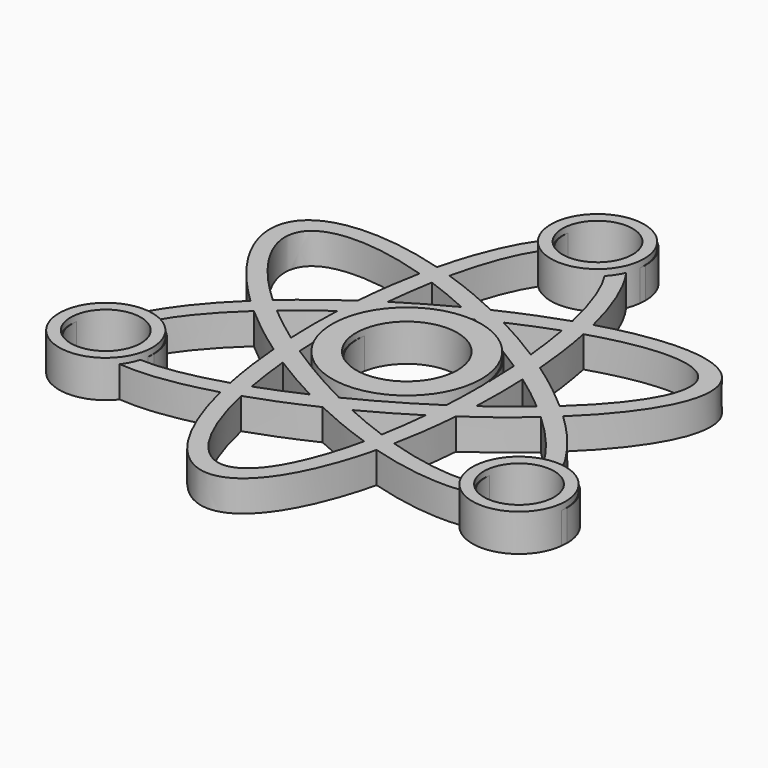
from build123d import *

# Parameters (mm, degrees)
F1_R     = 12
F1_R_2   = 8.15
F2_DEPTH = 6
F1_R_3   = 7.5
F1_R_4   = 5.65
F0_R     = 8.15
F0_R_2   = 5.65
F3_DEPTH = 5


with BuildPart() as f2:
    # F1 (on Top) → F2 (new body)
    with BuildSketch(Plane.XY):
        Circle(F1_R)
        Circle(F1_R_2, mode=Mode.SUBTRACT)
    extrude(amount=F2_DEPTH)


with BuildPart() as f2b:
    # F1 (on Top) → F2, piece 2 (new body)
    with BuildSketch(Plane.XY):
        with Locations((-33.1374317474, -19.1319051396)):
            Circle(F1_R_3)
        with Locations((-33.1374317474, -19.1319051396)):
            Circle(F1_R_4, mode=Mode.SUBTRACT)
    extrude(amount=F2_DEPTH)


with BuildPart() as f2c:
    # F1 (on Top) → F2, piece 3 (new body)
    with BuildSketch(Plane.XY):
        with Locations((33.5652192555, -19.3788883726)):
            Circle(F1_R_3)
        with Locations((33.5652192555, -19.3788883726)):
            Circle(F1_R_4, mode=Mode.SUBTRACT)
    extrude(amount=F2_DEPTH)


with BuildPart() as f2d:
    # F1 (on Top) → F2, piece 4 (new body)
    with BuildSketch(Plane.XY):
        with Locations((0.0270425226, 38.3360795677)):
            Circle(F1_R_3)
        with Locations((0.0270425226, 38.3360795677)):
            Circle(F1_R_4, mode=Mode.SUBTRACT)
    extrude(amount=F2_DEPTH)


with BuildPart() as f3:
    # F0 (on Top) → F3 (new body)
    with BuildSketch(Plane.XY):
        with BuildLine():
            add(Edge.make_bspline(
                [(-6.8281479501, 35.6153670276), (-10.3964562843, 30.7505631418), (-12.5794180407, 21.7881911761)],
                knots=[3.6142005533, 3.6142005533, 3.6142005533, 4.136351934, 4.136351934, 4.136351934], degree=2, weights=[1, 0.96611288, 1]))
            add(Edge.make_bspline(
                [(-12.5794180407, 21.7881911761), (-63.5959467611, 36.7171369819), (-25.1588360813, 0)],
                knots=[2.1468333731, 2.1468333731, 2.1468333731, 4.136351934, 4.136351934, 4.136351934], degree=2, weights=[1, 0.5447047794, 1]))
            add(Edge.make_bspline(
                [(-25.1588360813, 0), (-31.5395540563, -6.0951952888), (-34.0525181208, -11.4429254939)],
                knots=[5.2884260267, 5.2884260267, 5.2884260267, 5.7888730737, 5.7888730737, 5.7888730737], degree=2, weights=[1, 0.9688570969, 1]))
            ThreePointArc((-34.0525181208, -11.4429254939), (-32.6184418853, -11.398749972), (-31.2021943228, -11.6284649424))
            add(Edge.make_bspline(
                [(-23.0842721319, -1.9049402042), (-28.8407006291, -7.1898746007), (-31.2021943228, -11.6284649424)],
                knots=[5.3141014808, 5.3141014808, 5.3141014808, 5.8041996068, 5.8041996068, 5.8041996068], degree=2, weights=[1, 0.9701254233, 1]))
            add(Edge.make_bspline(
                [(-23.0842721319, -1.9049402042), (-19.2548852046, -5.2896457362), (-14.6603333228, -8.4641473903)],
                knots=[4.2163139158, 4.2163139158, 4.2163139158, 4.4991734706, 4.4991734706, 4.4991734706], degree=2, weights=[1, 0.9900154686, 1]))
            add(Edge.make_bspline(
                [(-14.6603333228, -8.4641473903), (-14.2084101868, -14.030396866), (-13.1918626754, -19.039095992)],
                knots=[4.9256044902, 4.9256044902, 4.9256044902, 5.208464045, 5.208464045, 5.208464045], degree=2, weights=[1, 0.9900154686, 1]))
            add(Edge.make_bspline(
                [(-25.9708285957, -21.1947915162), (-20.8855439548, -21.4568151153), (-13.1918626754, -19.039095992)],
                knots=[0.4639504735, 0.4639504735, 0.4639504735, 0.9690838264, 0.9690838264, 0.9690838264], degree=2, weights=[1, 0.968274225, 1]))
            ThreePointArc((-25.9708285957, -21.1947915162), (-26.5516990466, -22.5293003894), (-27.3793841564, -23.7264895026))
            add(Edge.make_bspline(
                [(-27.3793841564, -23.7264895026), (-21.3927870674, -24.3672437276), (-12.5794180407, -21.7881911761)],
                knots=[0.4748481149, 0.4748481149, 0.4748481149, 0.9947592804, 0.9947592804, 0.9947592804], degree=2, weights=[1, 0.966401396, 1]))
            add(Edge.make_bspline(
                [(-12.5794180407, -21.7881911761), (0, -73.4342739638), (12.5794180407, -21.7881911761)],
                knots=[5.2884260267, 5.2884260267, 5.2884260267, 7.2779445876, 7.2779445876, 7.2779445876], degree=2, weights=[1, 0.5447047794, 1]))
            add(Edge.make_bspline(
                [(12.5794180407, -21.7881911761), (21.6057072158, -24.429550463), (27.6471251634, -23.6959189871)],
                knots=[5.2884260267, 5.2884260267, 5.2884260267, 5.8203200725, 5.8203200725, 5.8203200725], degree=2, weights=[1, 0.9648440341, 1]))
            ThreePointArc((27.6471251634, -23.6959189871), (26.8931432652, -22.4926085087), (26.3794818209, -21.1687517449))
            add(Edge.make_bspline(
                [(13.1918626754, -19.039095992), (21.2208468241, -21.5621831608), (26.3794818209, -21.1687517449)],
                knots=[5.3141014808, 5.3141014808, 5.3141014808, 5.8402670021, 5.8402670021, 5.8402670021], degree=2, weights=[1, 0.9655928696, 1]))
            add(Edge.make_bspline(
                [(13.1918626754, -19.039095992), (14.2084101868, -14.030396866), (14.6603333228, -8.4641473903)],
                knots=[1.0747212622, 1.0747212622, 1.0747212622, 1.357580817, 1.357580817, 1.357580817], degree=2, weights=[1, 0.9900154686, 1]))
            add(Edge.make_bspline(
                [(14.6603333228, -8.4641473903), (19.2548852046, -5.2896457362), (23.0842721319, -1.9049402042)],
                knots=[1.7840118366, 1.7840118366, 1.7840118366, 2.0668713914, 2.0668713914, 2.0668713914], degree=2, weights=[1, 0.9900154686, 1]))
            add(Edge.make_bspline(
                [(31.3771657843, -11.9659434287), (29.0752743784, -7.4052350237), (23.0842721319, -1.9049402042)],
                knots=[0.4598507043, 0.4598507043, 0.4598507043, 0.9690838264, 0.9690838264, 0.9690838264], degree=2, weights=[1, 0.9677599453, 1]))
            ThreePointArc((31.3771657843, -11.9659434287), (32.7480265443, -11.6781030125), (34.1485023623, -11.6501958085))
            add(Edge.make_bspline(
                [(34.1485023623, -11.6501958085), (31.6718148928, -6.2215377523), (25.1588360813, 0)],
                knots=[0.4843791774, 0.4843791774, 0.4843791774, 0.9947592804, 0.9947592804, 0.9947592804], degree=2, weights=[1, 0.9676153386, 1]))
            add(Edge.make_bspline(
                [(25.1588360813, 0), (63.5959467611, 36.7171369819), (12.5794180407, 21.7881911761)],
                knots=[2.1468333731, 2.1468333731, 2.1468333731, 4.136351934, 4.136351934, 4.136351934], degree=2, weights=[1, 0.5447047794, 1]))
            add(Edge.make_bspline(
                [(12.5794180407, 21.7881911761), (10.4205252763, 30.6517454419), (6.9015425968, 35.5146251974)],
                knots=[2.1468333731, 2.1468333731, 2.1468333731, 2.6634816304, 2.6634816304, 2.6634816304], degree=2, weights=[1, 0.9668194548, 1]))
            ThreePointArc((6.9015425968, 35.5146251974), (6.2047415893, 34.2864574654), (5.2900837168, 33.210665386))
            add(Edge.make_bspline(
                [(9.8924094564, 20.9440361962), (8.1124850166, 28.9365653027), (5.2900837168, 33.210665386)],
                knots=[2.1725088272, 2.1725088272, 2.1725088272, 2.6850580062, 2.6850580062, 2.6850580062], degree=2, weights=[1, 0.9673410004, 1]))
            add(Edge.make_bspline(
                [(9.8924094564, 20.9440361962), (5.0464750177, 19.3200426022), (0, 16.9282947806)],
                knots=[4.2163139158, 4.2163139158, 4.2163139158, 4.4991734706, 4.4991734706, 4.4991734706], degree=2, weights=[1, 0.9900154686, 1]))
            add(Edge.make_bspline(
                [(0, 16.9282947806), (-5.0464750177, 19.3200426022), (-9.8924094564, 20.9440361962)],
                knots=[1.7840118366, 1.7840118366, 1.7840118366, 2.0668713914, 2.0668713914, 2.0668713914], degree=2, weights=[1, 0.9900154686, 1]))
            add(Edge.make_bspline(
                [(-5.2434979676, 33.2808277191), (-8.0967946137, 29.0070211038), (-9.8924094564, 20.9440361962)],
                knots=[3.5938067733, 3.5938067733, 3.5938067733, 4.11067648, 4.11067648, 4.11067648], degree=2, weights=[1, 0.9667911631, 1]))
            ThreePointArc((-5.2434979676, 33.2808277191), (-6.1465956187, 34.3729065668), (-6.8281479501, 35.6153670276))
        make_face()
        with BuildLine():
            add(Edge.make_bspline(
                [(-9.8924094564, -20.9440361962), (0, -65.364669311), (9.8924094564, -20.9440361962)],
                knots=[5.3141014808, 5.3141014808, 5.3141014808, 7.2522691336, 7.2522691336, 7.2522691336], degree=2, weights=[1, 0.5660550323, 1]))
            add(Edge.make_bspline(
                [(-9.8924094564, -20.9440361962), (-5.0464750177, -19.3200426022), (0, -16.9282947806)],
                knots=[1.0747212622, 1.0747212622, 1.0747212622, 1.357580817, 1.357580817, 1.357580817], degree=2, weights=[1, 0.9900154686, 1]))
            add(Edge.make_bspline(
                [(0, -16.9282947806), (5.0464750177, -19.3200426022), (9.8924094564, -20.9440361962)],
                knots=[4.9256044902, 4.9256044902, 4.9256044902, 5.208464045, 5.208464045, 5.208464045], degree=2, weights=[1, 0.9900154686, 1]))
        make_face(mode=Mode.SUBTRACT)
        with BuildLine():
            add(Edge.make_bspline(
                [(-11.500723238, -10.561649929), (-11.1183437103, -14.5201346451), (-10.4622745777, -18.1211911313)],
                knots=[5.0018649094, 5.0018649094, 5.0018649094, 5.2242056426, 5.2242056426, 5.2242056426], degree=2, weights=[1, 0.9938269364, 1]))
            add(Edge.make_bspline(
                [(-11.500723238, -10.561649929), (-7.5518465665, -13.0801819442), (-3.3962955254, -15.2407434505)],
                knots=[4.5951432057, 4.5951432057, 4.5951432057, 4.8296347551, 4.8296347551, 4.8296347551], degree=2, weights=[1, 0.9931345842, 1]))
            add(Edge.make_bspline(
                [(-10.4622745777, -18.1211911313), (-7.0156336139, -16.8888354237), (-3.3962955254, -15.2407434505)],
                knots=[1.0589796645, 1.0589796645, 1.0589796645, 1.2813203977, 1.2813203977, 1.2813203977], degree=2, weights=[1, 0.9938269364, 1]))
        make_face(mode=Mode.SUBTRACT)
        with BuildLine():
            add(Edge.make_bspline(
                [(-20.9245491554, 0), (-18.1339773242, -2.3687007785), (-14.8970187634, -4.6790935215)],
                knots=[4.2005723181, 4.2005723181, 4.2005723181, 4.4229130513, 4.4229130513, 4.4229130513], degree=2, weights=[1, 0.9938269364, 1]))
            add(Edge.make_bspline(
                [(-14.8970187634, 4.6790935215), (-18.1339773242, 2.3687007785), (-20.9245491554, 0)],
                knots=[5.0018649094, 5.0018649094, 5.0018649094, 5.2242056426, 5.2242056426, 5.2242056426], degree=2, weights=[1, 0.9938269364, 1]))
            add(Edge.make_bspline(
                [(-14.8970187634, 4.6790935215), (-15.1036931331, 0), (-14.8970187634, -4.6790935215)],
                knots=[4.5951432057, 4.5951432057, 4.5951432057, 4.8296347551, 4.8296347551, 4.8296347551], degree=2, weights=[1, 0.9931345842, 1]))
        make_face(mode=Mode.SUBTRACT)
        with BuildLine():
            add(Edge.make_bspline(
                [(-11.7950027096, -6.8098479895), (-6.1042800729, -10.5729232299), (0, -13.619695979)],
                knots=[4.527283772, 4.527283772, 4.527283772, 4.8974941888, 4.8974941888, 4.8974941888], degree=2, weights=[1, 0.9829168925, 1]))
            add(Edge.make_bspline(
                [(-11.7950027096, 6.8098479895), (-12.2085601458, 0), (-11.7950027096, -6.8098479895)],
                knots=[4.527283772, 4.527283772, 4.527283772, 4.8974941888, 4.8974941888, 4.8974941888], degree=2, weights=[1, 0.9829168925, 1]))
            add(Edge.make_bspline(
                [(-7.8378197498, 9.3081807072), (-9.8563553915, 8.0918074502), (-11.7950027096, 6.8098479895)],
                knots=[4.7700874936, 4.7700874936, 4.7700874936, 4.8974941888, 4.8974941888, 4.8974941888], degree=2, weights=[1, 0.9979716278, 1]))
            ThreePointArc((-7.8378197498, 9.3081807072), (-5.3517812773, -10.4755984452), (11.9981526935, -0.649200527))
            add(Edge.make_bspline(
                [(11.7950027096, -6.8098479895), (11.9804714737, -3.7558245831), (11.9981526935, -0.649200527)],
                knots=[1.3856911184, 1.3856911184, 1.3856911184, 1.5532494662, 1.5532494662, 1.5532494662], degree=2, weights=[1, 0.9964925773, 1]))
            add(Edge.make_bspline(
                [(0, -13.619695979), (6.1042800729, -10.5729232299), (11.7950027096, -6.8098479895)],
                knots=[1.3856911184, 1.3856911184, 1.3856911184, 1.7559015352, 1.7559015352, 1.7559015352], degree=2, weights=[1, 0.9829168925, 1]))
        make_face(mode=Mode.SUBTRACT)
        with Locations((0.0318146728, 0.2489945376)):
            Circle(F0_R, mode=Mode.SUBTRACT)
        with BuildLine():
            add(Edge.make_bspline(
                [(3.3962955254, -15.2407434505), (7.0156336139, -16.8888354237), (10.4622745777, -18.1211911313)],
                knots=[5.0018649094, 5.0018649094, 5.0018649094, 5.2242056426, 5.2242056426, 5.2242056426], degree=2, weights=[1, 0.9938269364, 1]))
            add(Edge.make_bspline(
                [(3.3962955254, -15.2407434505), (7.5518465665, -13.0801819442), (11.500723238, -10.561649929)],
                knots=[1.4535505521, 1.4535505521, 1.4535505521, 1.6880421015, 1.6880421015, 1.6880421015], degree=2, weights=[1, 0.9931345842, 1]))
            add(Edge.make_bspline(
                [(10.4622745777, -18.1211911313), (11.1183437103, -14.5201346451), (11.500723238, -10.561649929)],
                knots=[1.0589796645, 1.0589796645, 1.0589796645, 1.2813203977, 1.2813203977, 1.2813203977], degree=2, weights=[1, 0.9938269364, 1]))
        make_face(mode=Mode.SUBTRACT)
        with BuildLine():
            add(Edge.make_bspline(
                [(14.8970187634, -4.6790935215), (18.1339773242, -2.3687007785), (20.9245491554, 0)],
                knots=[1.8602722558, 1.8602722558, 1.8602722558, 2.0826129891, 2.0826129891, 2.0826129891], degree=2, weights=[1, 0.9938269364, 1]))
            add(Edge.make_bspline(
                [(14.8970187634, -4.6790935215), (15.1036931331, 0), (14.8970187634, 4.6790935215)],
                knots=[1.4535505521, 1.4535505521, 1.4535505521, 1.6880421015, 1.6880421015, 1.6880421015], degree=2, weights=[1, 0.9931345842, 1]))
            add(Edge.make_bspline(
                [(20.9245491554, 0), (18.1339773242, 2.3687007785), (14.8970187634, 4.6790935215)],
                knots=[1.0589796645, 1.0589796645, 1.0589796645, 1.2813203977, 1.2813203977, 1.2813203977], degree=2, weights=[1, 0.9938269364, 1]))
        make_face(mode=Mode.SUBTRACT)
        with BuildLine():
            add(Edge.make_bspline(
                [(-13.1918626754, 19.039095992), (-56.6074641333, 32.6823346555), (-23.0842721319, 1.9049402042)],
                knots=[2.1725088272, 2.1725088272, 2.1725088272, 4.11067648, 4.11067648, 4.11067648], degree=2, weights=[1, 0.5660550323, 1]))
            add(Edge.make_bspline(
                [(-13.1918626754, 19.039095992), (-14.2084101868, 14.030396866), (-14.6603333228, 8.4641473903)],
                knots=[4.2163139158, 4.2163139158, 4.2163139158, 4.4991734706, 4.4991734706, 4.4991734706], degree=2, weights=[1, 0.9900154686, 1]))
            add(Edge.make_bspline(
                [(-14.6603333228, 8.4641473903), (-19.2548852046, 5.2896457362), (-23.0842721319, 1.9049402042)],
                knots=[4.9256044902, 4.9256044902, 4.9256044902, 5.208464045, 5.208464045, 5.208464045], degree=2, weights=[1, 0.9900154686, 1]))
        make_face(mode=Mode.SUBTRACT)
        with BuildLine():
            add(Edge.make_bspline(
                [(0, 13.619695979), (-1.9292535333, 12.6567655398), (-3.8450407618, 11.6054901212)],
                knots=[4.527283772, 4.527283772, 4.527283772, 4.6455055558, 4.6455055558, 4.6455055558], degree=2, weights=[1, 0.9982534599, 1]))
            add(Edge.make_bspline(
                [(3.7462089914, 11.6596594984), (1.8793294581, 12.6816836809), (0, 13.619695979)],
                knots=[1.6407321764, 1.6407321764, 1.6407321764, 1.7559015352, 1.7559015352, 1.7559015352], degree=2, weights=[1, 0.9983424605, 1]))
            ThreePointArc((3.7462089914, 11.6596594984), (-0.0538123318, 12.2486890344), (-3.8450407618, 11.6054901212))
        make_face(mode=Mode.SUBTRACT)
        with BuildLine():
            add(Edge.make_bspline(
                [(-10.4622745777, 18.1211911313), (-11.1183437103, 14.5201346451), (-11.500723238, 10.561649929)],
                knots=[4.2005723181, 4.2005723181, 4.2005723181, 4.4229130513, 4.4229130513, 4.4229130513], degree=2, weights=[1, 0.9938269364, 1]))
            add(Edge.make_bspline(
                [(-3.3962955254, 15.2407434505), (-7.0156336139, 16.8888354237), (-10.4622745777, 18.1211911313)],
                knots=[1.8602722558, 1.8602722558, 1.8602722558, 2.0826129891, 2.0826129891, 2.0826129891], degree=2, weights=[1, 0.9938269364, 1]))
            add(Edge.make_bspline(
                [(-3.3962955254, 15.2407434505), (-7.5518465665, 13.0801819442), (-11.500723238, 10.561649929)],
                knots=[4.5951432057, 4.5951432057, 4.5951432057, 4.8296347551, 4.8296347551, 4.8296347551], degree=2, weights=[1, 0.9931345842, 1]))
        make_face(mode=Mode.SUBTRACT)
        with BuildLine():
            add(Edge.make_bspline(
                [(11.7950027096, 6.8098479895), (9.9536968222, 8.027438977), (8.0395831241, 9.1863120563)],
                knots=[1.3856911184, 1.3856911184, 1.3856911184, 1.5067166116, 1.5067166116, 1.5067166116], degree=2, weights=[1, 0.9981696624, 1]))
            add(Edge.make_bspline(
                [(11.9936285634, 1.2055552766), (11.9637542778, 4.0310984694), (11.7950027096, 6.8098479895)],
                knots=[1.6033846697, 1.6033846697, 1.6033846697, 1.7559015352, 1.7559015352, 1.7559015352], degree=2, weights=[1, 0.9970937345, 1]))
            ThreePointArc((11.9936285634, 1.2055552766), (10.7844503693, 5.5763602636), (8.0395831241, 9.1863120563))
        make_face(mode=Mode.SUBTRACT)
        with BuildLine():
            add(Edge.make_bspline(
                [(10.4622745777, 18.1211911313), (7.0156336139, 16.8888354237), (3.3962955254, 15.2407434505)],
                knots=[4.2005723181, 4.2005723181, 4.2005723181, 4.4229130513, 4.4229130513, 4.4229130513], degree=2, weights=[1, 0.9938269364, 1]))
            add(Edge.make_bspline(
                [(11.500723238, 10.561649929), (11.1183437103, 14.5201346451), (10.4622745777, 18.1211911313)],
                knots=[1.8602722558, 1.8602722558, 1.8602722558, 2.0826129891, 2.0826129891, 2.0826129891], degree=2, weights=[1, 0.9938269364, 1]))
            add(Edge.make_bspline(
                [(11.500723238, 10.561649929), (7.5518465665, 13.0801819442), (3.3962955254, 15.2407434505)],
                knots=[1.4535505521, 1.4535505521, 1.4535505521, 1.6880421015, 1.6880421015, 1.6880421015], degree=2, weights=[1, 0.9931345842, 1]))
        make_face(mode=Mode.SUBTRACT)
        with BuildLine():
            add(Edge.make_bspline(
                [(23.0842721319, 1.9049402042), (19.2548852046, 5.2896457362), (14.6603333228, 8.4641473903)],
                knots=[1.0747212622, 1.0747212622, 1.0747212622, 1.357580817, 1.357580817, 1.357580817], degree=2, weights=[1, 0.9900154686, 1]))
            add(Edge.make_bspline(
                [(14.6603333228, 8.4641473903), (14.2084101868, 14.030396866), (13.1918626754, 19.039095992)],
                knots=[1.7840118366, 1.7840118366, 1.7840118366, 2.0668713914, 2.0668713914, 2.0668713914], degree=2, weights=[1, 0.9900154686, 1]))
            add(Edge.make_bspline(
                [(23.0842721319, 1.9049402042), (56.6074641333, 32.6823346555), (13.1918626754, 19.039095992)],
                knots=[2.1725088272, 2.1725088272, 2.1725088272, 4.11067648, 4.11067648, 4.11067648], degree=2, weights=[1, 0.5660550323, 1]))
        make_face(mode=Mode.SUBTRACT)
        with BuildLine():
            ThreePointArc((7.5588571953, 38.5850741053), (-1.4572993615, 45.9302268808), (-6.8281479501, 35.6153670276))
            ThreePointArc((-6.8281479501, 35.6153670276), (-6.1465956187, 34.3729065668), (-5.2434979676, 33.2808277191))
            ThreePointArc((-5.2434979676, 33.2808277191), (0.008902124, 31.0852404744), (5.2900837168, 33.210665386))
            ThreePointArc((5.2900837168, 33.210665386), (6.2047415893, 34.2864574654), (6.9015425968, 35.5146251974))
            ThreePointArc((6.9015425968, 35.5146251974), (7.3926877262, 37.0150646326), (7.5588571953, 38.5850741053))
        make_face()
        with Locations((0.0588571953, 38.5850741053)):
            Circle(F0_R_2, mode=Mode.SUBTRACT)
        with BuildLine():
            ThreePointArc((-31.2021943228, -11.6284649424), (-32.6184418853, -11.398749972), (-34.0525181208, -11.4429254939))
            ThreePointArc((-34.0525181208, -11.4429254939), (-39.6959121723, -22.4631355286), (-27.3793841564, -23.7264895026))
            ThreePointArc((-27.3793841564, -23.7264895026), (-26.5516990466, -22.5293003894), (-25.9708285957, -21.1947915162))
            ThreePointArc((-25.9708285957, -21.1947915162), (-25.6974825729, -20.0531854433), (-25.6056170746, -18.882910602))
            ThreePointArc((-25.6056170746, -18.882910602), (-27.1673652006, -14.3017355692), (-31.2021943228, -11.6284649424))
        make_face()
        with Locations((-33.1056170746, -18.882910602)):
            Circle(F0_R_2, mode=Mode.SUBTRACT)
        with BuildLine():
            ThreePointArc((26.3794818209, -21.1687517449), (26.8931432652, -22.4926085087), (27.6471251634, -23.6959189871))
            ThreePointArc((27.6471251634, -23.6959189871), (36.0080175723, -26.2318061034), (41.0970339283, -19.129893835))
            ThreePointArc((41.0970339283, -19.129893835), (39.0918502699, -14.0252887207), (34.1485023623, -11.6501958085))
            ThreePointArc((34.1485023623, -11.6501958085), (32.7480265443, -11.6781030125), (31.3771657843, -11.9659434287))
            ThreePointArc((31.3771657843, -11.9659434287), (27.0061959333, -15.5506684267), (26.3794818209, -21.1687517449))
        make_face()
        with Locations((33.5970339283, -19.129893835)):
            Circle(F0_R_2, mode=Mode.SUBTRACT)
    extrude(amount=F3_DEPTH)


solid = Compound([f2.part, f2b.part, f2c.part, f2d.part, f3.part])
